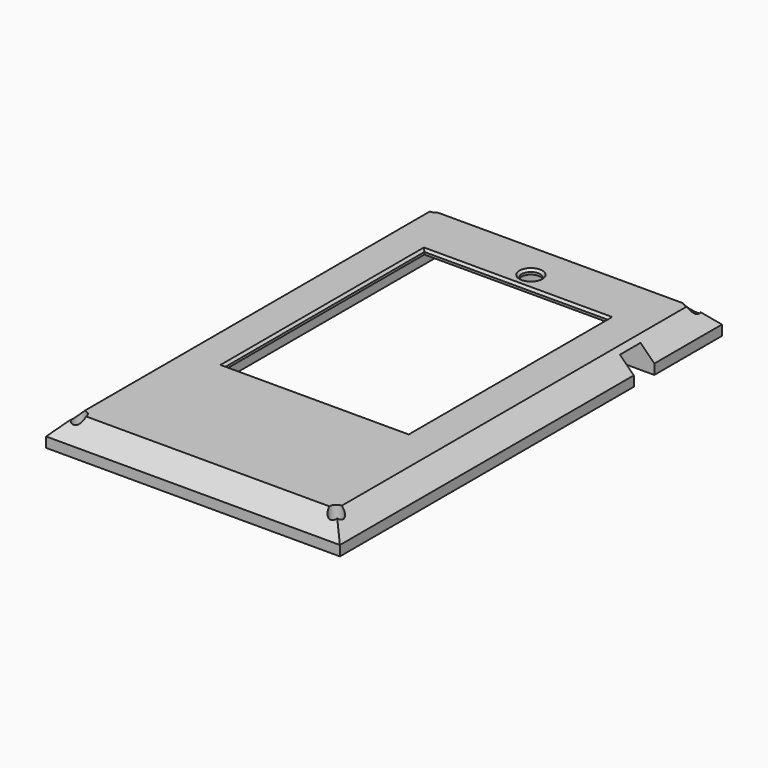
from build123d import *

# Parameters (mm, degrees)
F0_W        = 100
F0_H        = 136
F0_R        = 5
F0_R_2      = 3.75
F0_R_3      = 1.25
F0_W_2      = 12
F0_H_2      = 44
F1_DEPTH    = 15.5
F2_DEPTH    = 13
F4_R        = 3.75
F5_DEPTH    = 10
F6_T1_DEPTH = 211.4336597593
F6_T3_DEPTH = 311.4336597593
F7_SIZE     = 1.25
F8_SIZE     = 1.25
F9_W        = 12
F9_H        = 34
F9_W_2      = 20
F9_H_2      = 14
F10_DEPTH   = 13


# Not quite as in the source:
# - a fillet or chamfer that OpenCascade refuses, or shapes differently, is made with other operations: its cross-section is extruded or revolved along the edge and cut away or added


with BuildPart() as f1:
    # F0 (on Top) → F1 (new body)
    with BuildSketch(Plane.XY):
        Polygon((0, 196), (0, 0), (54, 0), (66, 0), (120, 0), (120, 196), align=None)
        with Locations((60, 108)):
            Rectangle(F0_W, F0_H, mode=Mode.SUBTRACT)
        with Locations((60, 186)):
            Circle(F0_R, mode=Mode.SUBTRACT)
        Polygon((54, 0), (0, 0), (0, 196), (120, 196), (120, 0), (66, 0), (66, -44), (140, -44), (140, 216), (-20, 216), (-20, -44), (54, -44), align=None)
        with Locations((-10, -34)):
            Circle(F0_R_2, mode=Mode.SUBTRACT)
        with Locations((130, -34)):
            Circle(F0_R_2, mode=Mode.SUBTRACT)
        with Locations((-10, 206)):
            Circle(F0_R_2, mode=Mode.SUBTRACT)
        with Locations((130, 206)):
            Circle(F0_R_2, mode=Mode.SUBTRACT)
        with Locations((130, -34)):
            Circle(F0_R_2)
        with Locations((130, -34)):
            Circle(F0_R_3, mode=Mode.SUBTRACT)
        with Locations((-10, -34)):
            Circle(F0_R_2)
        with Locations((-10, -34)):
            Circle(F0_R_3, mode=Mode.SUBTRACT)
        with Locations((-10, 206)):
            Circle(F0_R_2)
        with Locations((-10, 206)):
            Circle(F0_R_3, mode=Mode.SUBTRACT)
        with Locations((130, 206)):
            Circle(F0_R_2)
        with Locations((130, 206)):
            Circle(F0_R_3, mode=Mode.SUBTRACT)
        with Locations((60, -22)):
            Rectangle(F0_W_2, F0_H_2)
    extrude(amount=F1_DEPTH)

    # F0 (on Top) → F2 (cut)
    with BuildSketch(Plane.XY):
        Polygon((0, 196), (0, 0), (54, 0), (66, 0), (120, 0), (120, 196), align=None)
        with Locations((60, 108)):
            Rectangle(F0_W, F0_H, mode=Mode.SUBTRACT)
        with Locations((60, 186)):
            Circle(F0_R, mode=Mode.SUBTRACT)
    extrude(amount=F2_DEPTH, mode=Mode.SUBTRACT)

    # F4 (on offset) → F5 (cut)
    with BuildSketch(Plane.XY.offset(15.5)):
        with Locations((130, 208.356961264)):
            Circle(F4_R)
        with Locations((-10, 208.356961264)):
            Circle(F4_R)
        with Locations((130, -34)):
            Circle(F4_R)
        with Locations((-10, -34)):
            Circle(F4_R)
    extrude(amount=-F5_DEPTH, mode=Mode.SUBTRACT)

    # F6: chamfer of 10 on 4 edges, made by hand

    # F6_s2 → F6_t1 (cut)
    with BuildSketch(Plane.YZ.offset(-45.7168298797)):
        Polygon((216, 5.5), (206, 15.5), (216, 15.5), align=None)
        Polygon((-44, 5.5), (-34, 15.5), (-44, 15.5), align=None)
    extrude(amount=F6_T1_DEPTH, mode=Mode.SUBTRACT)

    # F6_s4 → F6_t3 (cut)
    with BuildSketch(Plane.XZ.offset(-241.7168298797)):
        Polygon((140, 5.5), (130, 15.5), (140, 15.5), align=None)
        Polygon((-10, 15.5), (-20, 5.5), (-20, 15.5), align=None)
    extrude(amount=F6_T3_DEPTH, mode=Mode.SUBTRACT)

    # F7
    f7_edges = [f1.edges().sort_by_distance(p)[0] for p in [
        (55, 186, 15.5),
    ]]
    chamfer(f7_edges, length=F7_SIZE)

    # F8
    f8_edges = [f1.edges().sort_by_distance(p)[0] for p in [
        (110, 108, 15.5),
        (60, 176, 15.5),
        (10, 108, 15.5),
        (60, 40, 15.5),
    ]]
    chamfer(f8_edges, length=F8_SIZE)

    # F9 (on face) → F10 (cut)
    with BuildSketch(Plane(origin=(0, 0, 0), x_dir=(1, 0, 0), z_dir=(0, 0, -1))):
        with Locations((60.329009831, 17)):
            Rectangle(F9_W, F9_H)
        with Locations((130, -163)):
            Rectangle(F9_W_2, F9_H_2)
    extrude(amount=-F10_DEPTH, mode=Mode.SUBTRACT)


solid = f1.part
